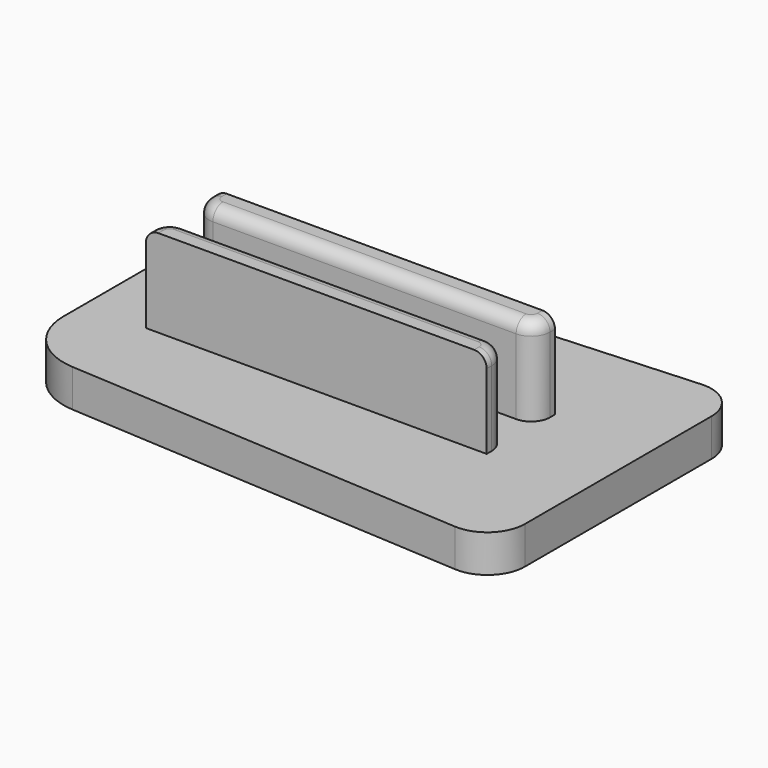
from build123d import *

# Parameters (mm, degrees)
F0_W     = 27.2240719226
F0_H     = 2
F1_DEPTH = 3
F2_DEPTH = 10
F3_R     = 1.5
F4_R     = 1
F5_R     = 3
F6_R     = 5


with BuildPart() as f1:
    # F0 (on Top) → F1 (new body)
    with BuildSketch(Plane.XY):
        Polygon((-7.7136544558, 22.5634722376), (-7.7136544558, 47.5634722376), (-47.7136544558, 45.1496791341), (-47.7136544558, 24.977265341), align=None)
        with Locations((-29.1016184945, 32.6534722376)):
            Rectangle(F0_W, F0_H, mode=Mode.SUBTRACT)
        with Locations((-29.1016184945, 37.4734722376)):
            Rectangle(F0_W, F0_H, mode=Mode.SUBTRACT)
    extrude(amount=F1_DEPTH)

    # F0 (on Top) → F2 (join)
    with BuildSketch(Plane.XY):
        with Locations((-29.1016184945, 32.6534722376)):
            Rectangle(F0_W, F0_H)
        with Locations((-29.1016184945, 37.4734722376)):
            Rectangle(F0_W, F0_H)
    extrude(amount=F2_DEPTH)

    # F3
    f3_edges = [f1.edges().sort_by_distance(p)[0] for p in [
        (-42.713654, 36.473472, 6.5),
        (-42.713654, 33.653472, 6.5),
        (-15.489583, 36.473472, 6.5),
        (-15.489583, 33.653472, 6.5),
    ]]
    fillet(f3_edges, radius=F3_R)

    # F4
    f4_edges = [f1.edges().sort_by_distance(p)[0] for p in [
        (-29.101618, 36.473472, 10),
        (-29.101618, 33.653472, 10),
        (-42.713654, 31.903472, 10),
        (-42.274315, 33.214132, 10),
        (-15.489583, 31.903472, 10),
        (-15.928922, 33.214132, 10),
        (-15.928922, 36.912812, 10),
        (-42.274315, 36.912812, 10),
        (-15.489583, 38.223472, 10),
        (-42.713654, 38.223472, 10),
    ]]
    fillet(f4_edges, radius=F4_R)

    # F5
    f5_edges = [f1.edges().sort_by_distance(p)[0] for p in [
        (-7.713654, 22.563472, 1.5),
        (-7.713654, 47.563472, 1.5),
    ]]
    fillet(f5_edges, radius=F5_R)

    # F6
    f6_edges = [f1.edges().sort_by_distance(p)[0] for p in [
        (-47.713654, 45.149679, 1.5),
        (-47.713654, 24.977265, 1.5),
    ]]
    fillet(f6_edges, radius=F6_R)


solid = f1.part
